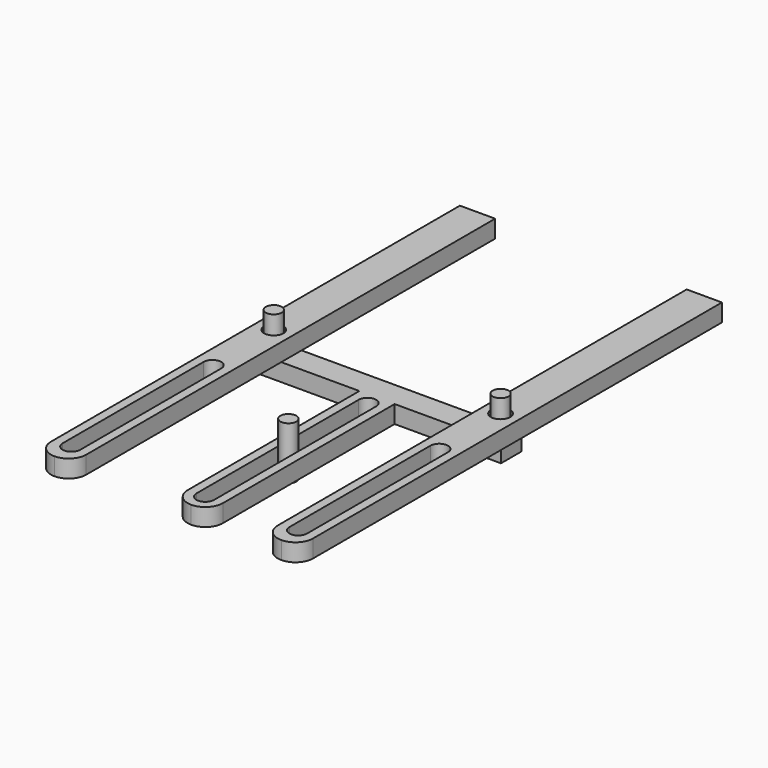
from build123d import *

# Parameters (mm, degrees)
F0_W      = 140.6747102737
F0_H      = 14.4206369296
F1_DEPTH  = 10
F2_R      = 4.5
F3_DEPTH  = 20
F4_W      = 16
F4_H      = 14.4206369296
F4_R      = 5.5
F5_DEPTH  = 10
F7_R      = 4.5
F8_DEPTH  = 15
F9_W      = 20
F9_H      = 131.7896815352
F10_DEPTH = 10
F11_R     = 9.99999
F12_R     = 9.99999
F13_R     = 9.99999


# Not quite as in the source:
# - a fillet or chamfer is up to 0.001 mm smaller than in the source, because OpenCascade refuses the exact size


with BuildPart() as f1:
    # F0 (on Top) → F1 (new body)
    with BuildSketch(Plane.XY):
        Rectangle(F0_W, F0_H)
    extrude(amount=-F1_DEPTH)

    # F2 (on face) → F3 (join)
    with BuildSketch(Plane.XY):
        with Locations((-64.3373551369, 0)):
            Circle(F2_R)
        with Locations((64.3373551369, 0)):
            Circle(F2_R)
    extrude(amount=F3_DEPTH)

    # F9 (on face) → F10 (join, through all)
    with BuildSketch(Plane.XY):
        with Locations((0, -73.1051592324)):
            Rectangle(F9_W, F9_H)
        with BuildLine():
            ThreePointArc((-5, -14), (0, -9), (5, -14))
            Line((5, -14), (5, -129))
            ThreePointArc((5, -129), (0, -134), (-5, -129))
            Line((-5, -129), (-5, -14))
        make_face(mode=Mode.SUBTRACT)
    extrude(amount=-F10_DEPTH)

    # F13 (radius 10 in the source; OpenCascade refuses exactly that, so slightly less here)
    f13_edges = [f1.edges().sort_by_distance(p)[0] for p in [
        (-10, -139, -5),
        (10, -139, -5),
    ]]
    fillet(f13_edges, radius=F13_R)


with BuildPart() as f5:
    # F4 (on face) → F5 (new body)
    with BuildSketch(Plane.XY):
        Polygon((-54.3373551369, 144.5), (-74.3373551369, 144.5), (-74.3373551369, -155.5), (-54.3373551369, -155.5), (-54.3373551369, -7.2103184648), (-70.3373551369, -7.2103184648), (-70.3373551369, 7.2103184648), (-54.3373551369, 7.2103184648), align=None)
        with BuildLine():
            ThreePointArc((-69.3373551369, -43.5), (-64.3373551369, -38.5), (-59.3373551369, -43.5))
            Line((-59.3373551369, -43.5), (-59.3373551369, -143.5))
            ThreePointArc((-59.3373551369, -143.5), (-64.3373551369, -148.5), (-69.3373551369, -143.5))
            Line((-69.3373551369, -143.5), (-69.3373551369, -43.5))
        make_face(mode=Mode.SUBTRACT)
        with Locations((-62.3373551369, 0)):
            Rectangle(F4_W, F4_H)
        with Locations((-64.3373551369, 0)):
            Circle(F4_R, mode=Mode.SUBTRACT)
    extrude(amount=F5_DEPTH)


with BuildPart() as f6_1:
    # F6: instance of F5
    add(f5.part.mirror(Plane.YZ))

    # F12 (radius 10 in the source; OpenCascade refuses exactly that, so slightly less here)
    f12_edges = [f6_1.edges().sort_by_distance(p)[0] for p in [
        (54.337355, -155.5, 5),
        (74.337355, -155.5, 5),
    ]]
    fillet(f12_edges, radius=F12_R)


with BuildPart() as f8:
    # F7 (on Top) → F8 (new body, symmetric)
    with BuildSketch(Plane.XY):
        with Locations((0, -70.0838316902)):
            Circle(F7_R)
    extrude(amount=F8_DEPTH, both=True)


with BuildPart() as f5_1:
    add(f5.part)

    # F11 (radius 10 in the source; OpenCascade refuses exactly that, so slightly less here)
    f11_edges = [f5_1.edges().sort_by_distance(p)[0] for p in [
        (-74.337355, -155.5, 5),
        (-54.337355, -155.5, 5),
    ]]
    fillet(f11_edges, radius=F11_R)


solid = Compound([f1.part, f6_1.part, f8.part, f5_1.part])
